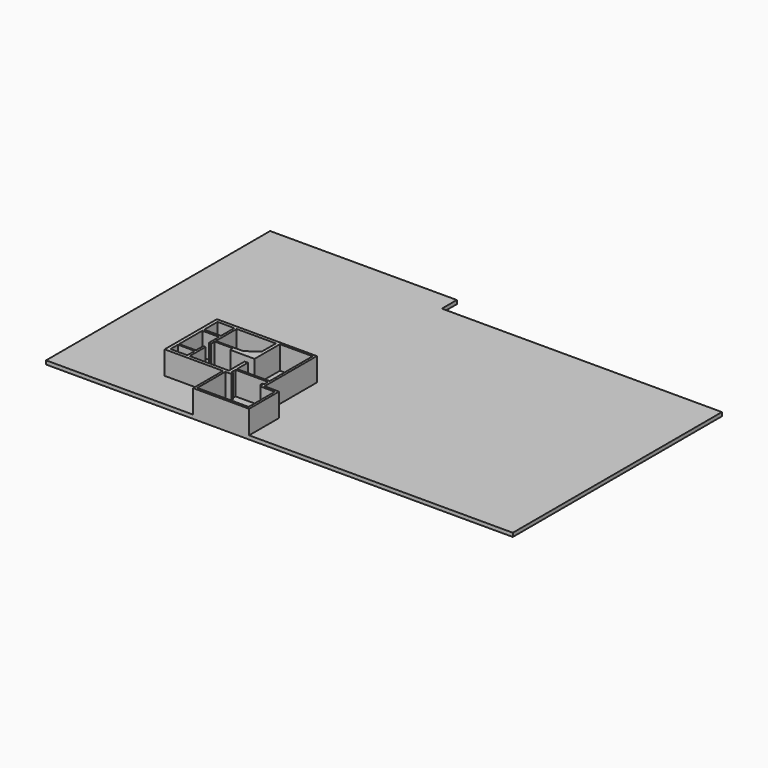
from build123d import *

# Parameters (mm, degrees)
F1_DEPTH = 400
F2_W     = 1800
F2_H     = 1000
F2_H_2   = 1800
F3_DEPTH = 2500


# Not quite as in the source:
# - a feature names something its author has since deleted; it is built from what else it names


with BuildPart() as f1:
    # F0 (on Top) → F1 (new body)
    with BuildSketch(Plane.XY):
        Polygon((-4996.7988580465, 16240.6410978539), (-24996.7988580465, 16240.6410978539), (-24996.7988580465, -13759.3589021461), (25003.2011419535, -13759.3589021461), (25003.2011419535, 14240.641097854), (-4996.7988580465, 14240.6410978539), align=None)
    extrude(amount=-F1_DEPTH)

    # F2 (on face) → F3 (join)
    with BuildSketch(Plane.XY):
        Polygon((-8546.7988580465, -2759.3589021461), (-15496.7988580465, -2759.3589021461), (-15496.7988580465, -9759.3589021461), (-9246.7988580465, -9759.3589021461), (-9246.7988580465, -13759.3589021461), (-3246.7988580465, -13759.3589021461), (-3246.7988580465, -9759.3589021461), (-4796.7988580465, -9759.3589021461), (-4796.7988580465, -3009.3589021461), (-4796.7988580465, -2759.3589021461), align=None)
        with Locations((-14246.7988580465, -8909.3589021461)):
            Rectangle(F2_W, F2_H, mode=Mode.SUBTRACT)
        Polygon((-8996.7988580465, -13509.3589021461), (-8996.7988580465, -9759.3589021461), (-8546.7988580465, -9759.3589021461), (-8346.7988580465, -9759.3589021461), (-8346.7988580465, -9509.3589021461), (-8546.7988580465, -9509.3589021461), (-8546.7988580465, -8959.3589021461), (-5046.7988580465, -8959.3589021461), (-5046.7988580465, -9509.3589021461), (-5246.7988580465, -9509.3589021461), (-5246.7988580465, -9759.3589021461), (-5046.7988580465, -9759.3589021461), (-5046.7988580465, -10009.3589021461), (-4796.7988580465, -10009.3589021461), (-3496.7988580465, -10009.3589021461), (-3496.7988580465, -13509.3589021461), align=None, mode=Mode.SUBTRACT)
        with Locations((-14246.7988580465, -4009.3589021461)):
            Rectangle(F2_W, F2_H_2, mode=Mode.SUBTRACT)
        Polygon((-8546.7988580465, -3009.3589021461), (-5046.7988580465, -3009.3589021461), (-5046.7988580465, -8759.3589021461), (-8546.7988580465, -8759.3589021461), (-8546.7988580465, -7309.3589021461), (-8896.7988580465, -7309.3589021461), (-8896.7988580465, -9409.3589021461), (-12196.7988580465, -9409.3589021461), (-13096.7988580465, -9409.3589021461), (-13096.7988580465, -8109.3589021461), (-13096.7988580465, -7286.1785888672), (-13346.7988580465, -7286.1785888672), (-13346.7988580465, -8259.3589021461), (-15146.7988580465, -8259.3589021461), (-15146.7988580465, -5159.3589021461), (-13346.7988580465, -5159.3589021461), (-13346.7988580465, -6521.4600563049), (-13096.7988580465, -6521.4600563049), (-13096.7988580465, -6049.3589021461), (-11146.7988580465, -6049.3589021461), (-11146.7988580465, -6409.3589021461), (-8896.7988580465, -6409.3589021461), (-8546.7988580465, -6409.3589021461), align=None, mode=Mode.SUBTRACT)
        Polygon((-8896.7988580465, -3109.3589021461), (-8896.7988580465, -5005.9270858765), (-10154.4055938721, -5899.3589021461), (-13096.7988580465, -5899.3589021461), (-13096.7988580465, -3109.3589021461), align=None, mode=Mode.SUBTRACT)
    extrude(amount=F3_DEPTH)


solid = f1.part
